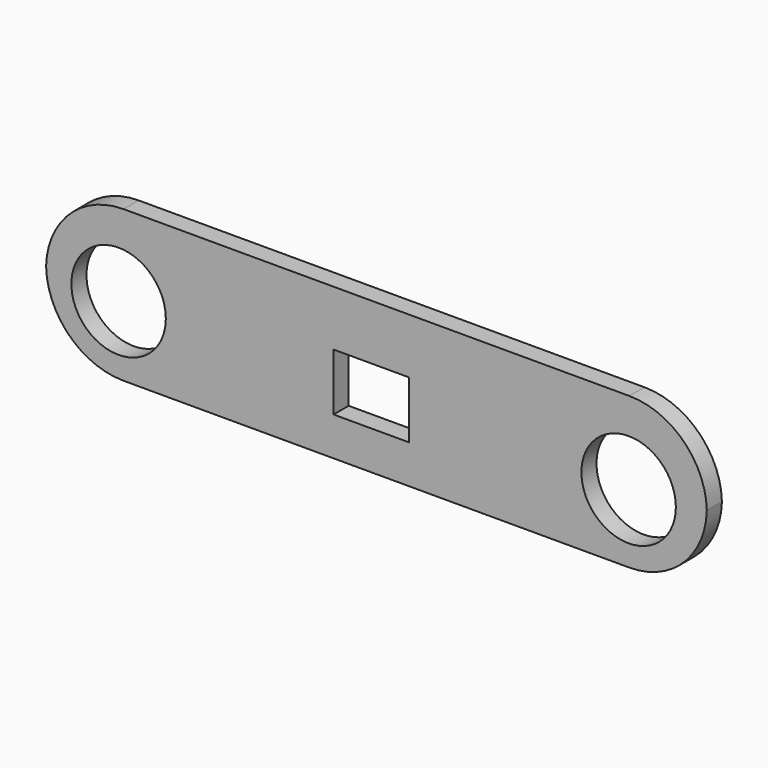
from build123d import *

# Parameters (mm, degrees)
F0_R        = 31.75
F0_W        = 50.8
F0_H        = 38.4544562548
F1_DEPTH    = 12.7
F2_T1_DEPTH = 273.2826573419
F2_T3_DEPTH = 273.264091489
F2_T5_DEPTH = 273.3012245177


# Not quite as in the source:
# - a fillet or chamfer that OpenCascade refuses, or shapes differently, is made with other operations: its cross-section is extruded or revolved along the edge and cut away or added


with BuildPart() as f1:
    # F0 (on Front) → F1 (new body)
    with BuildSketch(Plane.XZ):
        Polygon((248.1590109615, 55.626), (-196.0797500385, 55.626), (-196.0869890385, -45.974), (248.1590109615, -45.974), align=None)
        with Locations((-147.3189890385, 0)):
            Circle(F0_R, mode=Mode.SUBTRACT)
        with Locations((22.6070109615, -0.7874006405)):
            Rectangle(F0_W, F0_H, mode=Mode.SUBTRACT)
        with Locations((195.5810109615, 0)):
            Circle(F0_R, mode=Mode.SUBTRACT)
    extrude(amount=F1_DEPTH)

    # F2: fillet of radius 52.1165314684 on 4 edges, made by hand

    # F2_s2 → F2_t1 (cut)
    with BuildSketch(Plane.XZ.offset(-130.291328671)):
        with BuildLine():
            ThreePointArc((196.0424794931, 55.626), (232.8944323064, 40.3614213448), (248.1590109615, 3.5094685316))
            Line((248.1590109615, 3.5094685316), (248.1590109615, 55.626))
            Line((248.1590109615, 55.626), (196.0424794931, 55.626))
        make_face()
        with BuildLine():
            ThreePointArc((196.0424794931, -45.974), (232.8944323064, -30.7094213448), (248.1590109615, 6.1425314684))
            Line((248.1590109615, 6.1425314684), (248.1590109615, -45.974))
            Line((248.1590109615, -45.974), (196.0424794931, -45.974))
        make_face()
    extrude(amount=F2_T1_DEPTH, mode=Mode.SUBTRACT)

    # F2_s4 → F2_t3 (cut)
    with BuildSketch(Plane.XZ.offset(-130.2820457445)):
        with BuildLine():
            ThreePointArc((-143.9669317407, 55.626), (-180.8175716797, 40.3627341723), (-196.0834630768, 3.5131818345))
            Line((-196.0834630768, 3.5131818345), (-196.0797500385, 55.626))
            Line((-196.0797500385, 55.626), (-143.9669317407, 55.626))
        make_face()
    extrude(amount=F2_T3_DEPTH, mode=Mode.SUBTRACT)

    # F2_s6 → F2_t5 (cut)
    with BuildSketch(Plane.XZ.offset(-130.3006122588)):
        with BuildLine():
            ThreePointArc((-196.083275471, 6.1462447712), (-180.8200097756, -30.7081084706), (-143.9667441349, -45.974))
            Line((-143.9667441349, -45.974), (-196.0869890385, -45.974))
            Line((-196.0869890385, -45.974), (-196.083275471, 6.1462447712))
        make_face()
    extrude(amount=F2_T5_DEPTH, mode=Mode.SUBTRACT)


solid = f1.part
